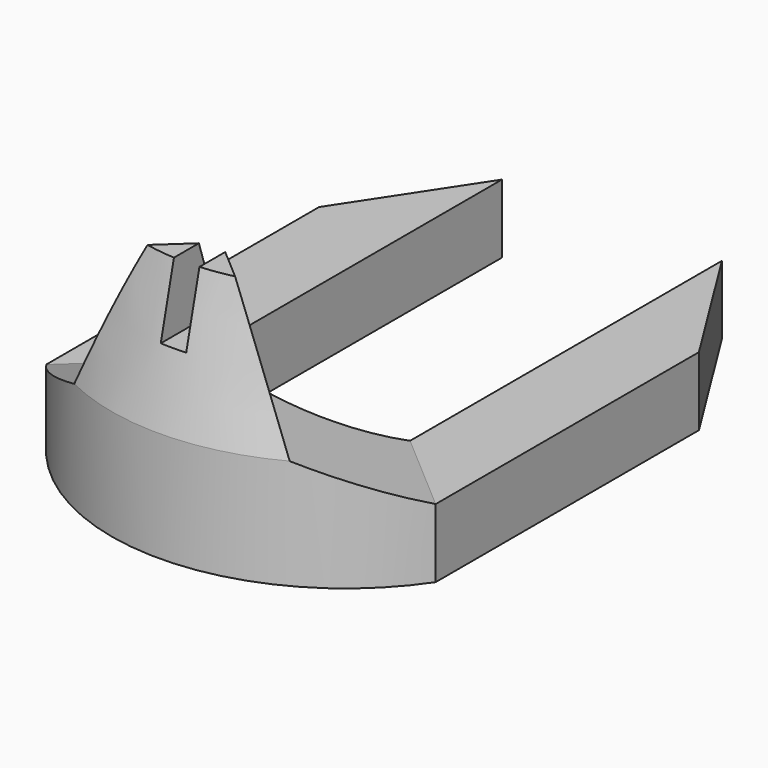
from build123d import *

# Parameters (mm, degrees)
F1_DEPTH    = 40
F2_DEPTH    = 25
F3_DEPTH    = 25
F4_SIZE2    = 41.212151
F4_SIZE     = 14.99999
F4_2_SIZE2  = 41.212151
F4_2_SIZE   = 14.99999
F5_DEPTH    = 25
F8_DEPTH    = 25
F9_T1_DEPTH = 305.3611948779
F9_T3_DEPTH = 305.3964050976
F9_T6_ANGLE = 198.1358920289
F9_T8_ANGLE = 199.0272584804


# Not quite as in the source:
# - a fillet or chamfer that OpenCascade refuses, or shapes differently, is made with other operations: its cross-section is extruded or revolved along the edge and cut away or added
# - a fillet or chamfer is up to 0.001 mm smaller than in the source, because OpenCascade refuses the exact size
# - ends of sketch curves that miss each other by under 0.0002 mm in the source are joined
# - a feature of the source that left no trace in its solid (it failed there, or was rolled back) is left out


with BuildPart() as f1:
    # F0 (on Top) → F1 (new body)
    with BuildSketch(Plane.XY):
        with BuildLine():
            Line((-40, -36.0045238119), (-70, -63.6819600925))
            ThreePointArc((-70, -63.6819600925), (0.5336536193, -99.3066602871), (70, -61.643119862))
            Line((70, -61.643119862), (40, -35.7918441296))
            ThreePointArc((40, -35.7918441296), (0.0635323292, -59.7960301521), (-40, -36.0045238119))
        make_face()
    extrude(amount=F1_DEPTH)

    # F0 (on Top) → F2 (join)
    with BuildSketch(Plane.XY):
        Polygon((-40, 105.9954761881), (-70, 60.3440771007), (-70, -63.6819600925), (-40, -36.0045238119), align=None)
    extrude(amount=F2_DEPTH)

    # F0 (on Top) → F3 (join)
    with BuildSketch(Plane.XY):
        Polygon((40, -35.7918441296), (70, -61.643119862), (70, 58.0248532689), (40, 105.9954761881), align=None)
    extrude(amount=F3_DEPTH)

    # F4 (size 15 and 41.2121612918 in the source; OpenCascade refuses exactly that, so slightly less here)
    f4_edges = [f1.edges().sort_by_distance(p)[0] for p in [
        (55, -48.717482, 40),
    ]]
    f4_side = f1.faces().sort_by_distance((55, -48.717482, 32.5))[0]
    chamfer(f4_edges, length=F4_SIZE, length2=F4_SIZE2, reference=f4_side)

    # F4#2 (size 15 and 41.2121612918 in the source; OpenCascade refuses exactly that, so slightly less here)
    f4_2_edges = [f1.edges().sort_by_distance(p)[0] for p in [
        (-55, -49.843242, 40),
    ]]
    f4_2_side = f1.faces().sort_by_distance((-55, -49.843242, 32.5))[0]
    chamfer(f4_2_edges, length=F4_2_SIZE, length2=F4_2_SIZE2, reference=f4_2_side)

    # F5 (add): a face of the model
    f5_faces = [f1.faces().sort_by_distance(p)[0] for p in [
        (0.2353529627, -82.8231732058, 40),
    ]]
    extrude(f5_faces, amount=F5_DEPTH)

    # F6 (on face) → F8 (join)
    with BuildSketch(Plane.XY.offset(65)):
        with BuildLine():
            Line((-4.7475561509, -99.219810589), (-4.7475561509, -59.5533930445))
            Line((-4.7475561509, -59.5533930445), (-38.3453534122, -90.5500754708))
            ThreePointArc((-38.3453534122, -90.5500754708), (-21.992530831, -96.6136201427), (-4.7475561509, -99.219810589))
        make_face()
        with BuildLine():
            Line((39.117860909, -89.4339641513), (4.4621424554, -59.5708130363))
            Line((4.4621424554, -59.5708130363), (4.4621283286, -99.1587323277))
            ThreePointArc((4.4621283286, -99.1587323277), (22.3094657758, -96.1475649652), (39.117860909, -89.4339641513))
        make_face()
    extrude(amount=F8_DEPTH)

    # F9: chamfer of 12 x 49.9835972411 on 4 edges, made by hand

    # F9_s2 → F9_t1 (cut)
    with BuildSketch(Plane(origin=(63.1741452332, 58.2832529798, 0), x_dir=(0, 0, 1), z_dir=(-0.73498516, -0.6780831915, 0))):
        Polygon((40.0164027589, -40.5516220902), (90, -52.5516220902), (90, -40.5516220902), align=None)
    extrude(amount=F9_T1_DEPTH, mode=Mode.SUBTRACT)

    # F9_s4 → F9_t3 (cut)
    with BuildSketch(Plane(origin=(165.0227982776, -142.2016620137, 0), x_dir=(0, 0, 1), z_dir=(-0.7575447308, 0.6527832572, 0))):
        Polygon((90, -54.2147436385), (40.0164027589, -42.2147436385), (90, -42.2147436385), align=None)
    extrude(amount=F9_T3_DEPTH, mode=Mode.SUBTRACT)

    # F9_s5 → F9_t6 (revolve, cut)
    with BuildSketch(Plane(origin=(-5.284270337, -12.1314567966, 0), x_dir=(0, 0, 1), z_dir=(0.3993440485, 0.9168011404, 0))):
        Polygon((90, -68.1975743243), (40.0164027589, -80.1975743243), (90, -80.1975743243), align=None)
    revolve(axis=Axis((-0.7068547451, -14.1253064914, 90), (0, 0, 1)), revolution_arc=F9_T6_ANGLE, mode=Mode.SUBTRACT)

    # F9_s7 → F9_t8 (revolve, cut)
    with BuildSketch(Plane(origin=(1.4990811594, -13.8871820878, 0), x_dir=(0, 0, 1), z_dir=(-0.1073236217, 0.9942241398, 0))):
        Polygon((40.0164027589, -87.4091372686), (90, -75.4091372686), (90, -87.4091372686), align=None)
    revolve(axis=Axis((-0.7068547451, -14.1253064914, 90), (0, 0, 1)), revolution_arc=F9_T8_ANGLE, mode=Mode.SUBTRACT)


solid = f1.part
